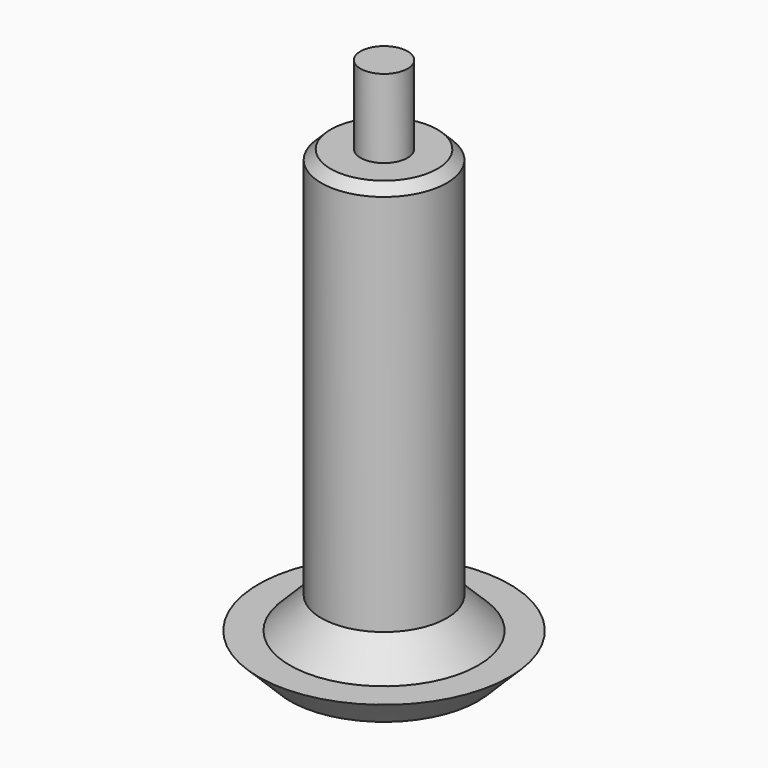
from build123d import *

# Parameters (mm, degrees)
F0_R     = 20
F1_DEPTH = 125
F2_R     = 7.5
F3_DEPTH = 25
F4_R     = 20
F5_DEPTH = 10
F5_TAPER = -45
F6_R     = 40
F6_R_2   = 30
F7_DEPTH = 10
F7_TAPER = 45
F8_SIZE2 = 3
F8_SIZE  = 3


with BuildPart() as f1:
    # F0 (on Top) → F1 (new body)
    with BuildSketch(Plane.XY):
        Circle(F0_R)
    extrude(amount=F1_DEPTH)

    # F2 (on face) → F3 (join)
    with BuildSketch(Plane.XY.offset(125)):
        Circle(F2_R)
    extrude(amount=F3_DEPTH)

    # F4 (on face) → F5 (join)
    with BuildSketch(Plane(origin=(0, 0, 0), x_dir=(1, 0, 0), z_dir=(0, 0, -1))):
        Circle(F4_R)
    extrude(amount=F5_DEPTH, taper=F5_TAPER)

    # F6 (on face) → F7 (join)
    with BuildSketch(Plane(origin=(0, 0, -10), x_dir=(1, 0, 0), z_dir=(0, 0, -1))):
        Circle(F6_R)
        Circle(F6_R_2, mode=Mode.SUBTRACT)
        Circle(F6_R_2)
    extrude(amount=F7_DEPTH, taper=F7_TAPER)

    # F8
    f8_edges = [f1.edges().sort_by_distance(p)[0] for p in [
        (-20, 0, 125),
    ]]
    chamfer(f8_edges, length=F8_SIZE, length2=F8_SIZE2)


solid = f1.part
